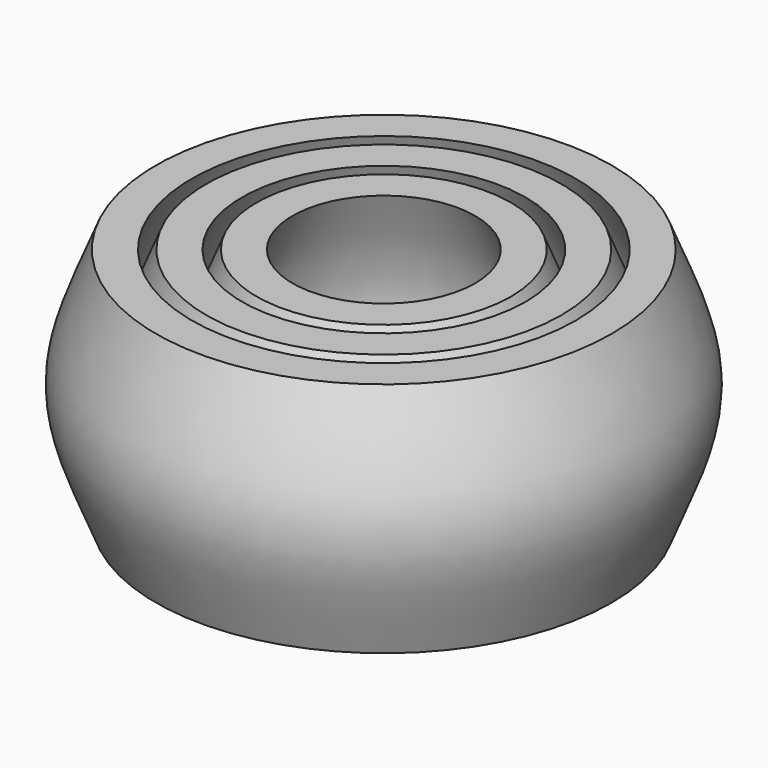
from build123d import *


# Not quite as in the source:
# - a feature names something its author has since deleted; it is built from what else it names


with BuildPart() as f1:
    # F0 (on Front) → F1 (revolve)
    with BuildSketch(Plane.XZ):
        with BuildLine():
            Line((13.5950473221, 3.0594923287), (17.3963618184, 3.0594923287))
            Line((17.3963618184, 3.0594923287), (17.3963618184, 15.575221673))
            add(Edge.make_bspline(
                [(13.5950473221, 3.0594923287), (15.5000473221, 7.292825662), (17.3963618184, 11.4340236675), (17.3963618184, 15.575221673)],
                knots=[0, 0, 0, 0, 0.5, 0.5, 0.5, 0.5], degree=3))
        make_face()
        with BuildLine():
            Line((17.3963618184, 15.575221673), (17.3963618184, 3.0594923287))
            add(Edge.make_bspline(
                [(17.3963618184, 3.0594923287), (18.9838618184, 7.292825662), (21.2063618184, 11.4340236675), (21.2063618184, 15.575221673)],
                knots=[0, 0, 0, 0, 0.5, 0.5, 0.5, 0.5], degree=3))
            Line((21.2063618184, 15.575221673), (17.3963618184, 15.575221673))
        make_face()
        with BuildLine():
            Line((17.3963618184, 28.0909510174), (17.3963618184, 15.575221673))
            Line((17.3963618184, 15.575221673), (21.2063618184, 15.575221673))
            add(Edge.make_bspline(
                [(21.2063618184, 15.575221673), (21.2063618184, 19.7164196785), (18.9838618184, 23.857617684), (17.3963618184, 28.0909510174)],
                knots=[0.5, 0.5, 0.5, 0.5, 1, 1, 1, 1], degree=3))
        make_face()
        with BuildLine():
            add(Edge.make_bspline(
                [(17.3963618184, 15.575221673), (17.3963618184, 19.7164196785), (15.5000473221, 23.857617684), (13.5950473221, 28.0909510174)],
                knots=[0.5, 0.5, 0.5, 0.5, 1, 1, 1, 1], degree=3))
            Line((17.3963618184, 15.575221673), (17.3963618184, 28.0909510174))
            Line((17.3963618184, 28.0909510174), (13.5950473221, 28.0909510174))
        make_face()
    revolve(axis=Axis((3.9369999431, 0, 18.5394347056), (0, 0, 1)))


with BuildPart() as f1b:
    # F0 (on Front) → F1, piece 2 (revolve)
    with BuildSketch(Plane.XZ):
        with BuildLine():
            add(Edge.make_bspline(
                [(22.7216763147, 15.575221673), (22.6830307897, 19.7201419856), (20.8270694931, 23.8538228515), (18.9203618184, 28.0909510174)],
                knots=[0.4995517914, 0.4995517914, 0.4995517914, 0.4995517914, 1, 1, 1, 1], degree=3))
            Line((22.7216763147, 15.575221673), (22.7216763147, 28.0909510174))
            Line((22.7216763147, 28.0909510174), (18.9203618184, 28.0909510174))
        make_face()
        with BuildLine():
            Line((22.7216763147, 15.575221673), (26.5316763147, 15.575221673))
            add(Edge.make_bspline(
                [(26.5316763147, 15.575221673), (26.5316763147, 19.7164196785), (24.3091763147, 23.857617684), (22.7216763147, 28.0909510174)],
                knots=[0.5, 0.5, 0.5, 0.5, 1, 1, 1, 1], degree=3))
            Line((22.7216763147, 28.0909510174), (22.7216763147, 15.575221673))
        make_face()
        with BuildLine():
            Line((22.7216763147, 15.309013096), (22.7216763147, 3.0594923287))
            add(Edge.make_bspline(
                [(22.7216763147, 3.0594923287), (24.3091763147, 7.292825662), (26.5316763147, 11.4340236675), (26.5316763147, 15.575221673)],
                knots=[0, 0, 0, 0, 0.5, 0.5, 0.5, 0.5], degree=3))
            Line((26.5316763147, 15.575221673), (22.7216763147, 15.575221673))
            add(Edge.make_bspline(
                [(22.7216763147, 15.309013096), (22.7224980817, 15.3977548969), (22.7225036042, 15.4864908603), (22.7216763147, 15.575221673)],
                knots=[0.4888386358, 0.4888386358, 0.4888386358, 0.4888386358, 0.4995517914, 0.4995517914, 0.4995517914, 0.4995517914], degree=3))
        make_face()
        with BuildLine():
            Line((19.084725447, 3.0594923287), (22.7216763147, 3.0594923287))
            Line((22.7216763147, 3.0594923287), (22.7216763147, 15.309013096))
            add(Edge.make_bspline(
                [(19.084725447, 3.0594923287), (20.9472006495, 7.1983261121), (22.684179292, 11.2597467075), (22.7216763147, 15.309013096)],
                knots=[0, 0, 0, 0, 0.4888386358, 0.4888386358, 0.4888386358, 0.4888386358], degree=3))
        make_face()
    revolve(axis=Axis((3.9369999431, 0, 18.5394347056), (0, 0, 1)))


with BuildPart() as f1c:
    # F0 (on Front) → F1, piece 3 (revolve)
    with BuildSketch(Plane.XZ):
        with BuildLine():
            add(Edge.make_bspline(
                [(24.2456763147, 3.0594923287), (26.1506763147, 7.292825662), (28.0469908111, 11.4340236675), (28.0469908111, 15.575221673)],
                knots=[0, 0, 0, 0, 0.5, 0.5, 0.5, 0.5], degree=3))
            Line((24.2456763147, 3.0594923287), (28.0469908111, 3.0594923287))
            Line((28.0469908111, 3.0594923287), (28.0469908111, 15.575221673))
        make_face()
        with BuildLine():
            add(Edge.make_bspline(
                [(28.0469908111, 15.575221673), (28.0469908111, 19.7164196785), (26.1506763147, 23.857617684), (24.2456763147, 28.0909510174)],
                knots=[0.5, 0.5, 0.5, 0.5, 1, 1, 1, 1], degree=3))
            Line((28.0469908111, 15.575221673), (28.0469908111, 28.0909510174))
            Line((28.0469908111, 28.0909510174), (24.2456763147, 28.0909510174))
        make_face()
        with BuildLine():
            Line((28.0469908111, 15.575221673), (28.0469908111, 3.0594923287))
            add(Edge.make_bspline(
                [(28.0469908111, 3.0594923287), (29.6344908111, 7.292825662), (31.8569908111, 11.4340236675), (31.8569908111, 15.575221673)],
                knots=[0, 0, 0, 0, 0.5, 0.5, 0.5, 0.5], degree=3))
            Line((31.8569908111, 15.575221673), (28.0469908111, 15.575221673))
        make_face()
        with BuildLine():
            Line((28.0469908111, 28.0909510174), (28.0469908111, 15.575221673))
            Line((28.0469908111, 15.575221673), (31.8569908111, 15.575221673))
            add(Edge.make_bspline(
                [(31.8569908111, 15.575221673), (31.8569908111, 19.7164196785), (29.6344908111, 23.857617684), (28.0469908111, 28.0909510174)],
                knots=[0.5, 0.5, 0.5, 0.5, 1, 1, 1, 1], degree=3))
        make_face()
    revolve(axis=Axis((3.9369999431, 0, 18.5394347056), (0, 0, 1)))


solid = Compound([f1.part, f1b.part, f1c.part])
